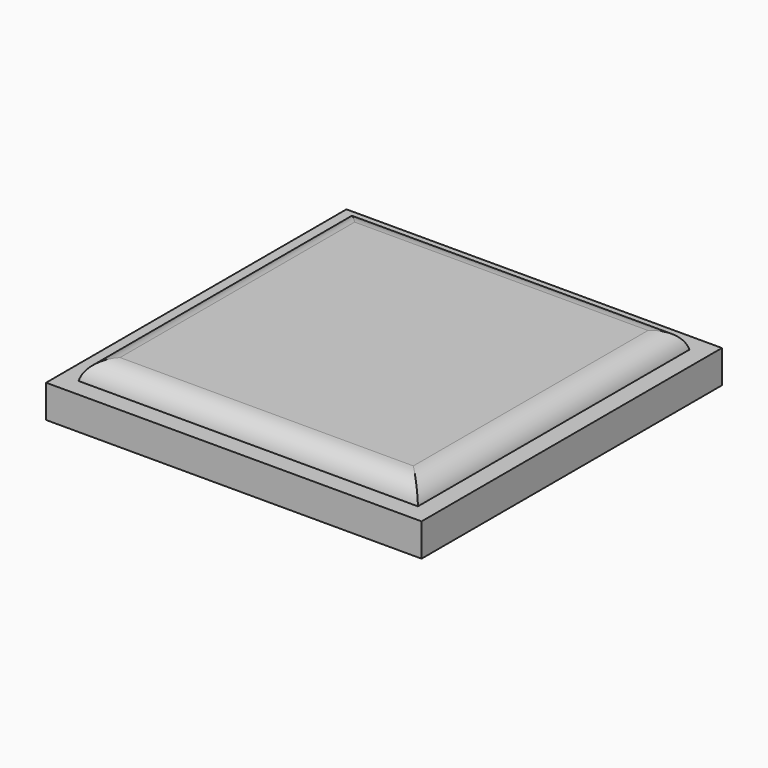
from build123d import *

# Parameters (mm, degrees)
F2_W     = 80
F2_H     = 80
F2_W_2   = 72
F2_H_2   = 72
F3_DEPTH = 3.5
F4_W     = 72.5
F4_H     = 72.5
F5_DEPTH = 7.5
F6_R     = 5


with BuildPart() as f3:
    # F2 (on Top) → F3 (new body, symmetric)
    with BuildSketch(Plane.XY):
        Rectangle(F2_W, F2_H)
        Rectangle(F2_W_2, F2_H_2, mode=Mode.SUBTRACT)
    extrude(amount=F3_DEPTH, both=True)


with BuildPart() as f5:
    # F4 (on Top) → F5 (new body, symmetric)
    with BuildSketch(Plane.XY):
        Rectangle(F4_W, F4_H)
    extrude(amount=F5_DEPTH, both=True)

    # F6
    f6_edges = [f5.edges().sort_by_distance(p)[0] for p in [
        (0, -36.25, 7.5),
        (36.25, 0, 7.5),
        (0, 36.25, 7.5),
        (-36.25, 0, 7.5),
        (0, -36.25, -7.5),
        (36.25, 0, -7.5),
        (0, 36.25, -7.5),
        (-36.25, 0, -7.5),
    ]]
    fillet(f6_edges, radius=F6_R)


with BuildPart() as f7_1:
    # F7: copy of F3
    add(f3.part)


with BuildPart() as f5_1:
    add(f5.part)

    # F8: cut F7_1
    add(f7_1.part, mode=Mode.SUBTRACT)


solid = Compound([f3.part, f5_1.part])
